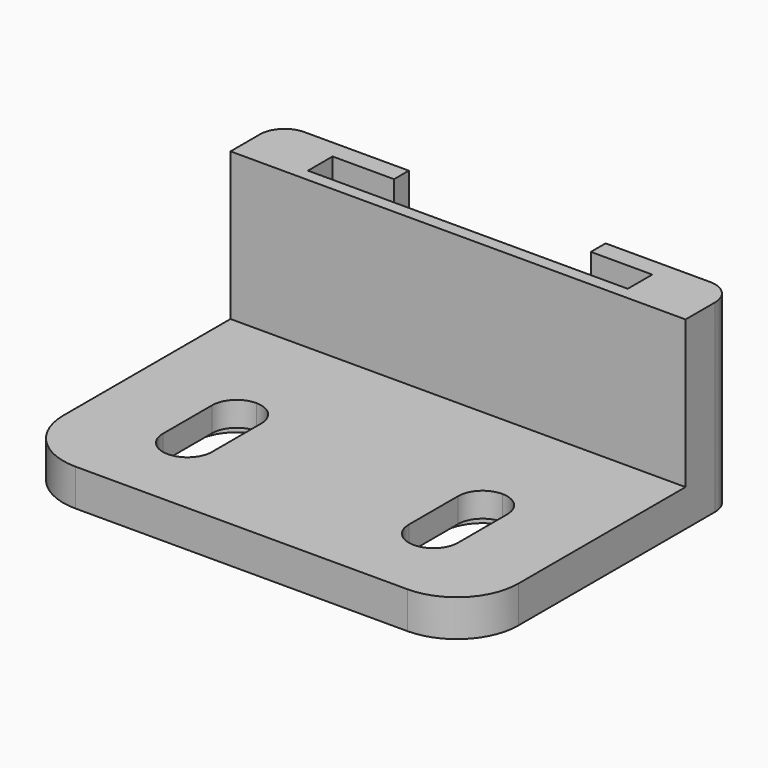
from build123d import *

# Parameters (mm, degrees)
F0_W        = 16
F0_H        = 22
F0_W_2      = 4
F0_H_2      = 9
F1_DEPTH    = 3
F2_DEPTH    = 15
F3_DEPTH    = 2.5
F4_DEPTH    = 2.5
F5_T1_DEPTH = 3
F5_T3_DEPTH = 25
F7_W        = 4
F7_H        = 9
F8_DEPTH    = 1
F10_DEPTH   = 1
F11_R       = 5


# Not quite as in the source:
# - a fillet or chamfer that OpenCascade refuses, or shapes differently, is made with other operations: its cross-section is extruded or revolved along the edge and cut away or added
# - two fillets or chamfers of one size are made in one step


with BuildPart() as f1:
    # F0 (on Top) → F1 (new body)
    with BuildSketch(Plane.XY):
        with Locations((8, 11)):
            Rectangle(F0_W, F0_H)
        with Locations((6, 9.5)):
            Rectangle(F0_W_2, F0_H_2, mode=Mode.SUBTRACT)
        with Locations((24, 11)):
            Rectangle(F0_W, F0_H)
        with Locations((26, 9.5)):
            Rectangle(F0_W_2, F0_H_2, mode=Mode.SUBTRACT)
    extrude(amount=F1_DEPTH)

    # F0 (on Top) → F2 (join)
    with BuildSketch(Plane.XY):
        Polygon((0, 27), (0, 23), (3, 23), (3, 25.5), (8, 25.5), (8, 27), align=None)
        Polygon((0, 23), (0, 22), (16, 22), (16, 23), (3, 23), align=None)
        Polygon((16, 23), (16, 22), (32, 22), (32, 23), (29, 23), align=None)
        Polygon((29, 23), (32, 23), (32, 27), (24, 27), (24, 25.5), (29, 25.5), align=None)
    extrude(amount=F2_DEPTH)

    # F3 (add): a face of the model
    f3_faces = [f1.faces().sort_by_distance(p)[0] for p in [
        (32, 0.3088689042, 1.5),
    ]]
    extrude(f3_faces, amount=F3_DEPTH)

    # F4 (add): a face of the model
    f4_faces = [f1.faces().sort_by_distance(p)[0] for p in [
        (0, 0.3088689042, 1.5),
    ]]
    extrude(f4_faces, amount=F4_DEPTH)

    # F5: fillet of radius 2 on 10 edges, made by hand

    # F5_s2 → F5_t1 (join)
    with BuildSketch(Plane.XY):
        with BuildLine():
            ThreePointArc((28, 12), (27.4142135624, 13.4142135624), (26, 14))
            Line((26, 14), (28, 14))
            Line((28, 14), (28, 12))
        make_face()
        with BuildLine():
            ThreePointArc((28, 7), (27.4142135624, 5.5857864376), (26, 5))
            Line((26, 5), (28, 5))
            Line((28, 5), (28, 7))
        make_face()
        with BuildLine():
            ThreePointArc((26, 14), (24.5857864376, 13.4142135624), (24, 12))
            Line((24, 12), (24, 14))
            Line((24, 14), (26, 14))
        make_face()
        with BuildLine():
            ThreePointArc((24, 7), (24.5857864376, 5.5857864376), (26, 5))
            Line((26, 5), (24, 5))
            Line((24, 5), (24, 7))
        make_face()
        with BuildLine():
            ThreePointArc((8, 12), (7.4142135624, 13.4142135624), (6, 14))
            Line((6, 14), (8, 14))
            Line((8, 14), (8, 12))
        make_face()
        with BuildLine():
            ThreePointArc((8, 7), (7.4142135624, 5.5857864376), (6, 5))
            Line((6, 5), (8, 5))
            Line((8, 5), (8, 7))
        make_face()
        with BuildLine():
            ThreePointArc((6, 14), (4.5857864376, 13.4142135624), (4, 12))
            Line((4, 12), (4, 14))
            Line((4, 14), (6, 14))
        make_face()
        with BuildLine():
            ThreePointArc((4, 7), (4.5857864376, 5.5857864376), (6, 5))
            Line((6, 5), (4, 5))
            Line((4, 5), (4, 7))
        make_face()
    extrude(amount=F5_T1_DEPTH)

    # F5_s4 → F5_t3 (cut)
    with BuildSketch(Plane.XY.offset(-5)):
        with BuildLine():
            ThreePointArc((32.5, 27), (33.9142135624, 26.4142135624), (34.5, 25))
            Line((34.5, 25), (34.5, 27))
            Line((34.5, 27), (32.5, 27))
        make_face()
        with BuildLine():
            ThreePointArc((-0.5, 27), (-1.9142135624, 26.4142135624), (-2.5, 25))
            Line((-2.5, 25), (-2.5, 27))
            Line((-2.5, 27), (-0.5, 27))
        make_face()
    extrude(amount=F5_T3_DEPTH, mode=Mode.SUBTRACT)

    # F7 (on face) → F8 (cut)
    with BuildSketch(Plane.XY):
        with BuildLine():
            Line((2.7, 12), (2.7, 7))
            ThreePointArc((2.7000000011, 7), (6, 3.7000000011), (9.2999999989, 7))
            Line((9.3, 7), (9.3, 12))
            ThreePointArc((9.3, 12), (6, 15.3), (2.7, 12))
        make_face()
        with Locations((6, 9.5)):
            Rectangle(F7_W, F7_H, mode=Mode.SUBTRACT)
        with Locations((6, 9.5)):
            Rectangle(F7_W, F7_H)
    extrude(amount=F8_DEPTH, mode=Mode.SUBTRACT)

    # F9 (on face) → F10 (cut)
    with BuildSketch(Plane.XY):
        with BuildLine():
            Line((22.7, 12), (22.7, 7))
            ThreePointArc((22.7, 7), (26, 3.7), (29.3, 7))
            Line((29.3, 7), (29.3, 12))
            ThreePointArc((29.3, 12), (26, 15.3), (22.7, 12))
        make_face()
    extrude(amount=F10_DEPTH, mode=Mode.SUBTRACT)

    # F11
    f11_edges = [f1.edges().sort_by_distance(p)[0] for p in [
        (34.5, 0, 1.5),
        (-2.5, 0, 1.5),
    ]]
    fillet(f11_edges, radius=F11_R)


solid = f1.part
